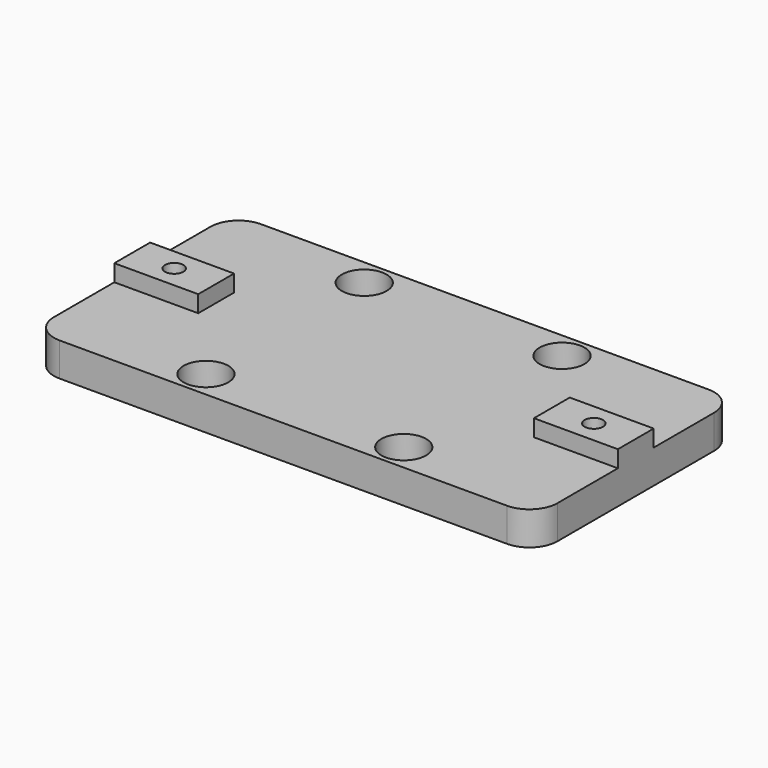
from build123d import *

# Parameters (mm, degrees)
F0_R     = 4
F0_R_2   = 1.65
F0_R_3   = 2
F1_DEPTH = 6
F2_DEPTH = 5
F3_DEPTH = 3


# Not quite as in the source:
# - a feature names something its author has since deleted; it is built from what else it names


with BuildPart() as f1:
    # F0 (on Top) → F1 (new body)
    with BuildSketch(Plane.XY):
        with BuildLine():
            Line((40, 22.5), (-40, 22.5))
            ThreePointArc((-40, 22.5), (-43.5355339059, 21.0355339059), (-45, 17.5))
            Line((-45, 17.5), (-45, 4))
            Line((-45, 4), (-30, 4))
            Line((-30, 4), (-30, 0))
            Line((-30, 0), (-30, -4))
            Line((-30, -4), (-45, -4))
            Line((-45, -4), (-45, -17.5))
            ThreePointArc((-45, -17.5), (-43.5355339059, -21.0355339059), (-40, -22.5))
            Line((-40, -22.5), (40, -22.5))
            ThreePointArc((40, -22.5), (43.5355339059, -21.0355339059), (45, -17.5))
            Line((45, -17.5), (45, -4))
            Line((45, -4), (30, -4))
            Line((30, -4), (30, 0))
            Line((30, 0), (30, 4))
            Line((30, 4), (45, 4))
            Line((45, 4), (45, 17.5))
            ThreePointArc((45, 17.5), (43.5355339059, 21.0355339059), (40, 22.5))
        make_face()
        with Locations((-17.6776695297, -17.6776695297)):
            Circle(F0_R, mode=Mode.SUBTRACT)
        with Locations((17.6776695297, -17.6776695297)):
            Circle(F0_R, mode=Mode.SUBTRACT)
        with Locations((-17.6776695297, 17.6776695297)):
            Circle(F0_R, mode=Mode.SUBTRACT)
        with Locations((17.6776695297, 17.6776695297)):
            Circle(F0_R, mode=Mode.SUBTRACT)
        Polygon((-30, 4), (-45, 4), (-45, -4), (-30, -4), (-30, 0), align=None)
        with Locations((-37.5, 0)):
            Circle(F0_R_2, mode=Mode.SUBTRACT)
        Polygon((45, -4), (45, 4), (30, 4), (30, 0), (30, -4), align=None)
        with Locations((37.5, 0)):
            Circle(F0_R_2, mode=Mode.SUBTRACT)
        with Locations((-17.6776695297, 17.6776695297)):
            Circle(F0_R)
        with Locations((-17.6776695297, 17.6776695297)):
            Circle(F0_R_2, mode=Mode.SUBTRACT)
        with Locations((-17.6776695297, -17.6776695297)):
            Circle(F0_R)
        with Locations((-17.6776695297, -17.6776695297)):
            Circle(F0_R_3, mode=Mode.SUBTRACT)
        with Locations((17.6776695297, 17.6776695297)):
            Circle(F0_R)
        with Locations((17.6776695297, 17.6776695297)):
            Circle(F0_R_3, mode=Mode.SUBTRACT)
        with Locations((17.6776695297, -17.6776695297)):
            Circle(F0_R)
        with Locations((17.6776695297, -17.6776695297)):
            Circle(F0_R_3, mode=Mode.SUBTRACT)
    extrude(amount=-F1_DEPTH)

    # F0 (on Top) → F2 (cut)
    with BuildSketch(Plane.XY):
        with Locations((-17.6776695297, 17.6776695297)):
            Circle(F0_R)
        with Locations((-17.6776695297, 17.6776695297)):
            Circle(F0_R_2, mode=Mode.SUBTRACT)
        with Locations((-17.6776695297, 17.6776695297)):
            Circle(F0_R_2)
        with Locations((-17.6776695297, -17.6776695297)):
            Circle(F0_R)
        with Locations((-17.6776695297, -17.6776695297)):
            Circle(F0_R_3, mode=Mode.SUBTRACT)
        with Locations((17.6776695297, -17.6776695297)):
            Circle(F0_R)
        with Locations((17.6776695297, -17.6776695297)):
            Circle(F0_R_3, mode=Mode.SUBTRACT)
        with Locations((17.6776695297, 17.6776695297)):
            Circle(F0_R)
        with Locations((17.6776695297, 17.6776695297)):
            Circle(F0_R_3, mode=Mode.SUBTRACT)
    extrude(amount=-F2_DEPTH, mode=Mode.SUBTRACT)

    # F0 (on Top) → F3 (join)
    with BuildSketch(Plane.XY):
        Polygon((-30, 4), (-45, 4), (-45, -4), (-30, -4), (-30, 0), align=None)
        with Locations((-37.5, 0)):
            Circle(F0_R_2, mode=Mode.SUBTRACT)
        Polygon((45, -4), (45, 4), (30, 4), (30, 0), (30, -4), align=None)
        with Locations((37.5, 0)):
            Circle(F0_R_2, mode=Mode.SUBTRACT)
    extrude(amount=F3_DEPTH)


solid = f1.part
